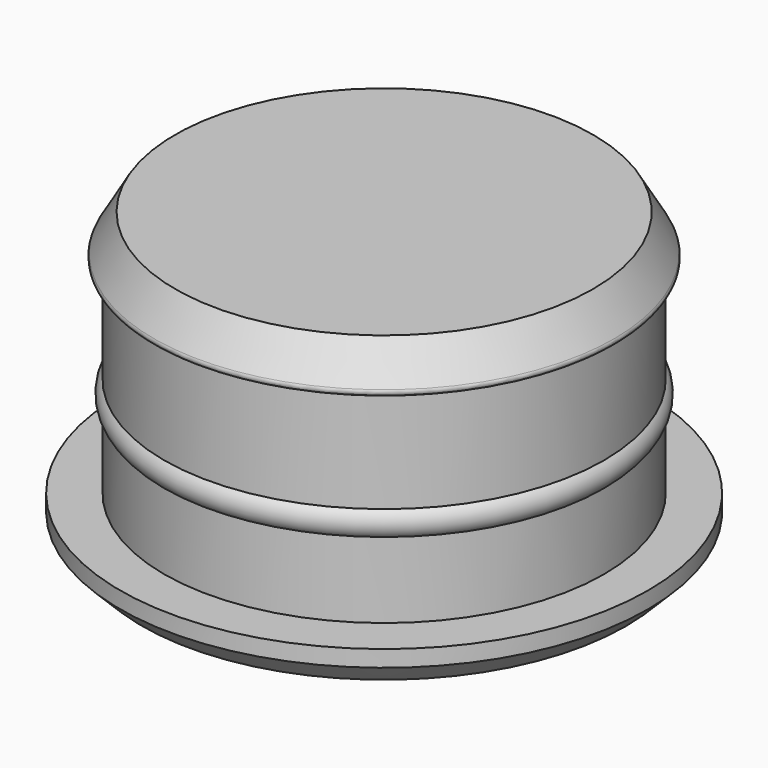
from build123d import *

# Parameters (mm, degrees)
F2_SIZE  = 2
F3_SIZE2 = 1.49999
F3_SIZE  = 0.69999
F4_R     = 0.4


# Not quite as in the source:
# - a fillet or chamfer is up to 0.001 mm smaller than in the source, because OpenCascade refuses the exact size


with BuildPart() as f1:
    # F0 (on Front) → F1 (revolve)
    with BuildSketch(Plane.XZ):
        with BuildLine():
            Line((0, 26), (0, 0))
            Line((0, 0), (24, 0))
            Line((24, 0), (24, 3.5))
            Line((24, 3.5), (20, 3.5))
            Line((20, 3.5), (20, 10.3819660113))
            ThreePointArc((20, 10.3819660113), (20.5, 11.5), (20, 12.6180339887))
            Line((20, 12.6180339887), (20, 21.7))
            Line((20, 21.7), (21.5, 21.7))
            Line((21.5, 21.7), (19, 26))
            Line((19, 26), (0, 26))
        make_face()
    revolve(axis=Axis((0, 0, 13), (0, 0, 1)))

    # F2
    f2_edges = [f1.edges().sort_by_distance(p)[0] for p in [
        (-24, 0, 0),
    ]]
    chamfer(f2_edges, length=F2_SIZE)

    # F3 (size 0.7 and 1.5 in the source; OpenCascade refuses exactly that, so slightly less here)
    f3_edges = [f1.edges().sort_by_distance(p)[0] for p in [
        (-21.5, 0, 21.7),
    ]]
    f3_side = f1.faces().sort_by_distance((-20.25, 0, 23.85))[0]
    chamfer(f3_edges, length=F3_SIZE, length2=F3_SIZE2, reference=f3_side)

    # F4
    f4_edges = [f1.edges().sort_by_distance(p)[0] for p in [
        (-21.148171, 0, 22.305146),
    ]]
    fillet(f4_edges, radius=F4_R)


solid = f1.part
